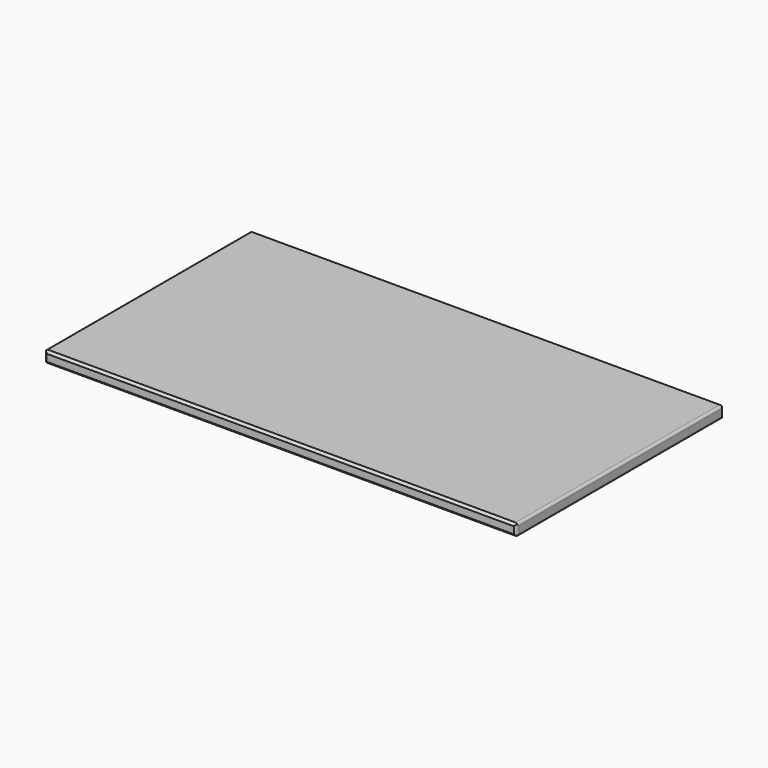
from build123d import *

# Parameters (mm, degrees)
F0_W        = 1000
F0_H        = 550
F1_DEPTH    = 25
F2_SIZE     = 5
F3_SIZE     = 5
F4_T1_DEPTH = 565
F4_T3_DEPTH = 35.3553390593
F5_T1_DEPTH = 565
F5_T3_DEPTH = 35.3553390593
F6_R        = 3
F7_DEPTH    = 12
F8_R        = 3
F9_DEPTH    = 12
F10_R       = 3
F11_DEPTH   = 12
F12_R       = 3
F13_DEPTH   = 12


# Not quite as in the source:
# - a fillet or chamfer that OpenCascade refuses, or shapes differently, is made with other operations: its cross-section is extruded or revolved along the edge and cut away or added


with BuildPart() as f1:
    # F0 (on Top) → F1 (new body)
    with BuildSketch(Plane.XY):
        Rectangle(F0_W, F0_H)
    extrude(amount=F1_DEPTH)

    # F2
    f2_edges = [f1.edges().sort_by_distance(p)[0] for p in [
        (-500, -275, 12.5),
        (500, -275, 12.5),
        (0, -275, 0),
        (0, -275, 25),
    ]]
    chamfer(f2_edges, length=F2_SIZE)

    # F3
    f3_edges = [f1.edges().sort_by_distance(p)[0] for p in [
        (500, 275, 12.5),
        (-500, 275, 12.5),
        (0, 275, 0),
        (0, 275, 25),
    ]]
    chamfer(f3_edges, length=F3_SIZE)

    # F4: fillet of radius 5 on 4 edges, made by hand

    # F4_s2 → F4_t1 (cut)
    with BuildSketch(Plane.XZ.offset(-282.5)):
        with BuildLine():
            ThreePointArc((-500, 5), (-498.5355339059, 1.4644660941), (-495, 0))
            Line((-495, 0), (-500, 0))
            Line((-500, 0), (-500, 5))
        make_face()
        with BuildLine():
            ThreePointArc((-500, 20), (-498.5355339059, 23.5355339059), (-495, 25))
            Line((-495, 25), (-500, 25))
            Line((-500, 25), (-500, 20))
        make_face()
    extrude(amount=F4_T1_DEPTH, mode=Mode.SUBTRACT)

    # F4_s4 → F4_t3 (cut)
    with BuildSketch(Plane.XY.offset(-5.1776695297)):
        with BuildLine():
            ThreePointArc((-500, 267.9289321881), (-499.6193976626, 269.84234935), (-498.5355339059, 271.4644660941))
            Line((-498.5355339059, 271.4644660941), (-500, 270))
            Line((-500, 270), (-500, 267.9289321881))
        make_face()
        with BuildLine():
            ThreePointArc((-500, -267.9289321881), (-499.6193976626, -269.84234935), (-498.5355339059, -271.4644660941))
            Line((-498.5355339059, -271.4644660941), (-500, -270))
            Line((-500, -270), (-500, -267.9289321881))
        make_face()
    extrude(amount=F4_T3_DEPTH, mode=Mode.SUBTRACT)

    # F5: fillet of radius 5 on 4 edges, made by hand

    # F5_s2 → F5_t1 (cut)
    with BuildSketch(Plane.XZ.offset(-282.5)):
        with BuildLine():
            ThreePointArc((495, 0), (498.5355339059, 1.4644660941), (500, 5))
            Line((500, 5), (500, 0))
            Line((500, 0), (495, 0))
        make_face()
        with BuildLine():
            ThreePointArc((495, 25), (498.5355339059, 23.5355339059), (500, 20))
            Line((500, 20), (500, 25))
            Line((500, 25), (495, 25))
        make_face()
    extrude(amount=F5_T1_DEPTH, mode=Mode.SUBTRACT)

    # F5_s4 → F5_t3 (cut)
    with BuildSketch(Plane.XY.offset(-5.1776695297)):
        with BuildLine():
            ThreePointArc((498.5355339059, 271.4644660941), (499.6193976626, 269.84234935), (500, 267.9289321881))
            Line((500, 267.9289321881), (500, 270))
            Line((500, 270), (498.5355339059, 271.4644660941))
        make_face()
        with BuildLine():
            ThreePointArc((500, -267.9289321881), (499.6193976626, -269.84234935), (498.5355339059, -271.4644660941))
            Line((498.5355339059, -271.4644660941), (500, -270))
            Line((500, -270), (500, -267.9289321881))
        make_face()
    extrude(amount=F5_T3_DEPTH, mode=Mode.SUBTRACT)

    # F6 (on face) → F7 (cut)
    with BuildSketch(Plane(origin=(0, 0, 0), x_dir=(1, 0, 0), z_dir=(0, 0, -1))):
        with Locations((470, 245)):
            Circle(F6_R)
    extrude(amount=-F7_DEPTH, mode=Mode.SUBTRACT)

    # F8 (on face) → F9 (cut)
    with BuildSketch(Plane(origin=(0, 0, 0), x_dir=(1, 0, 0), z_dir=(0, 0, -1))):
        with Locations((470, -245)):
            Circle(F8_R)
    extrude(amount=-F9_DEPTH, mode=Mode.SUBTRACT)

    # F10 (on face) → F11 (cut)
    with BuildSketch(Plane(origin=(0, 0, 0), x_dir=(1, 0, 0), z_dir=(0, 0, -1))):
        with Locations((-470, 245)):
            Circle(F10_R)
    extrude(amount=-F11_DEPTH, mode=Mode.SUBTRACT)

    # F12 (on face) → F13 (cut)
    with BuildSketch(Plane(origin=(0, 0, 0), x_dir=(1, 0, 0), z_dir=(0, 0, -1))):
        with Locations((-470, -245)):
            Circle(F12_R)
    extrude(amount=-F13_DEPTH, mode=Mode.SUBTRACT)


solid = f1.part
